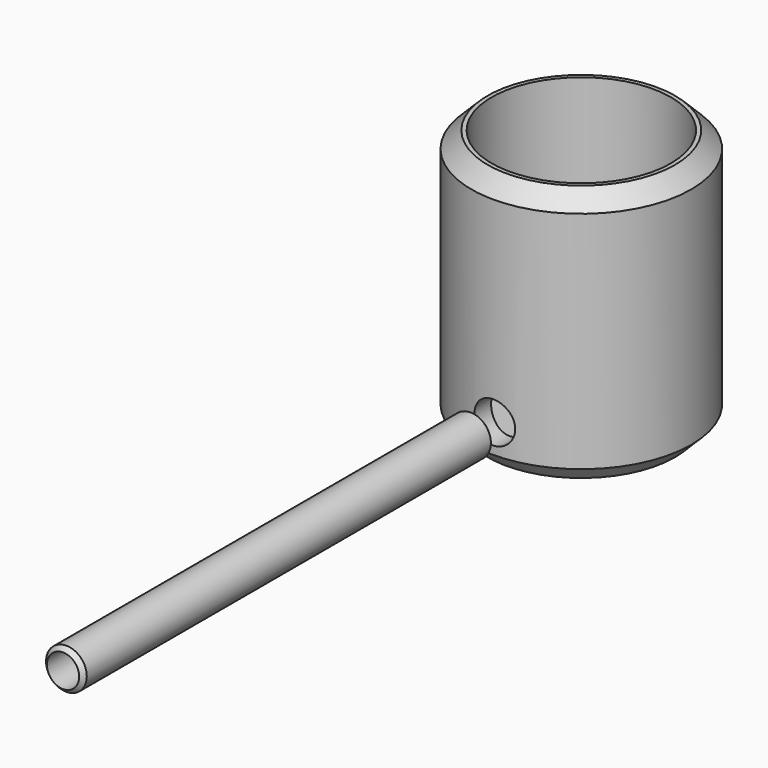
from build123d import *

# Parameters (mm, degrees)
F0_W      = 34.29
F0_H      = 80.2478848061
F5_T      = -6.35
F4_R      = 6.35
F6_DEPTH  = 165.1
F12_R     = 6.35
F7_DEPTH  = 165.1
F8_R      = 5.0354944202
F13_DEPTH = 237.491
F14_DEPTH = 72.3910001
F16_SIZE  = 5.08
F11_SIZE  = 5.08


# Not quite as in the source:
# - a fillet or chamfer that OpenCascade refuses, or shapes differently, is made with other operations: its cross-section is extruded or revolved along the edge and cut away or added


with BuildPart() as f2:
    # F0 (on Front) → F2 (revolve)
    with BuildSketch(Plane.XZ):
        with Locations((17.145, 0)):
            Rectangle(F0_W, F0_H)
    revolve(axis=Axis((0, 0, -6.2726922333), (0, 0, -1)))

    # F5
    f5_openings = [f2.faces().sort_by_distance(p)[0] for p in [
        (0, 0, 40.123942),
    ]]
    offset(amount=F5_T, openings=f5_openings)


with BuildPart() as f6:
    # F4 (on offset) → F6 (new body)
    with BuildSketch(Plane.XZ.offset(38.1)):
        with Locations((0, -12.0859783907)):
            Circle(F4_R)
    extrude(amount=F6_DEPTH)


with BuildPart() as f7:
    # F12 (on offset) → F7 (new body)
    with BuildSketch(Plane.XZ.offset(38.1)):
        with Locations((0, -26.1077899699)):
            Circle(F12_R)
    extrude(amount=F7_DEPTH)


with BuildPart() as f13_tool:
    # F8 (on face) → F13 (new body, through all)
    with BuildSketch(Plane.XZ.offset(203.2)):
        with Locations((0, -26.1077899699)):
            Circle(F8_R)
    extrude(amount=-F13_DEPTH)


with BuildPart() as f2_1:
    add(f2.part)

    # F13: cut by f13_tool
    add(f13_tool.part, mode=Mode.SUBTRACT)

    # F12 (on offset) → F14 (cut, through all)
    with BuildSketch(Plane.XZ.offset(38.1)):
        with Locations((0, -26.1077899699)):
            Circle(F12_R)
    extrude(amount=-F14_DEPTH, mode=Mode.SUBTRACT)

    # F16
    f16_edges = [f2_1.edges().sort_by_distance(p)[0] for p in [
        (-34.29, 0, 40.123942),
    ]]
    chamfer(f16_edges, length=F16_SIZE)

    # F11
    f11_edges = [f2_1.edges().sort_by_distance(p)[0] for p in [
        (-34.29, 0, -40.123942),
    ]]
    chamfer(f11_edges, length=F11_SIZE)


with BuildPart() as f7_1:
    add(f7.part)

    # F13: cut by f13_tool
    add(f13_tool.part, mode=Mode.SUBTRACT)

    # F10: chamfer of 2.54 on 1 edges, made by hand

    # F10_s1 → F10_t2 (revolve, cut)
    with BuildSketch(Plane.XY.offset(-26.1077899699)):
        Polygon((6.35, -200.66), (3.81, -203.2), (6.35, -203.2), align=None)
    revolve(axis=Axis((0, -203.2, -26.1077899699), (0, -1, 0)), mode=Mode.SUBTRACT)

    # F15: chamfer of 5.08 on 1 edges, made by hand

    # F15_s1 → F15_t2 (revolve, cut)
    with BuildSketch(Plane.XY.offset(-26.1077899699)):
        Polygon((6.35, -43.18), (1.27, -38.1), (6.35, -38.1), align=None)
    revolve(axis=Axis((0, -38.1, -26.1077899699), (0, -1, 0)), mode=Mode.SUBTRACT)


solid = Compound([f2_1.part, f7_1.part])
